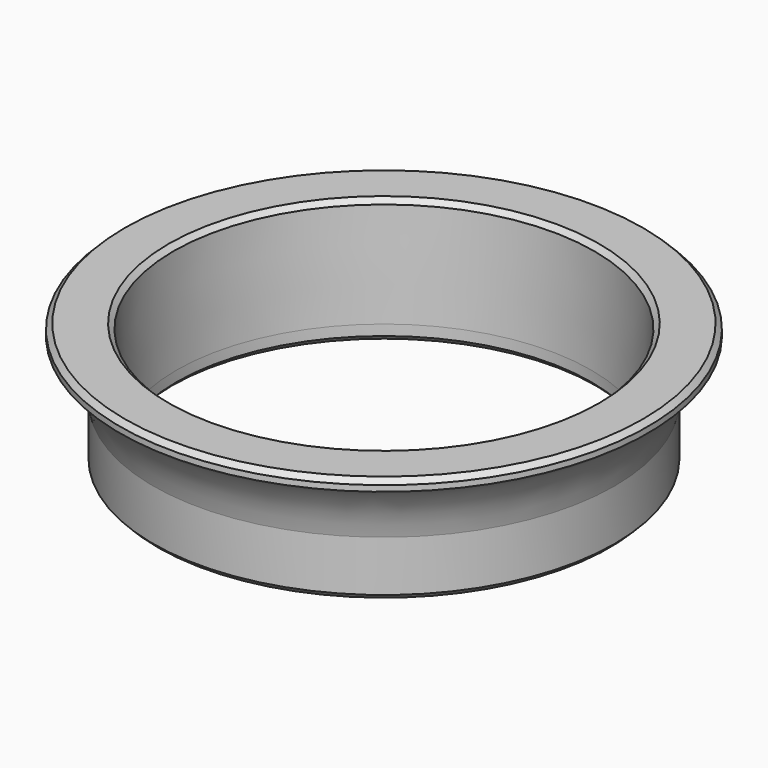
from build123d import *


# Not quite as in the source:
# - a fillet or chamfer that OpenCascade refuses, or shapes differently, is made with other operations: its cross-section is extruded or revolved along the edge and cut away or added


with BuildPart() as f1:
    # F0 (on Front) → F1 (revolve)
    with BuildSketch(Plane.XZ):
        with BuildLine():
            Line((-74.5, 17.9942867992), (-74.5, 0))
            Line((-74.5, 0), (-67, 0))
            Line((-67, 0), (-66.9277426788, 0))
            Line((-66.9277426788, 0), (-66.9277426788, 5))
            Line((-66.9277426788, 5), (-68, 39.9997837721))
            Line((-68, 39.9997837721), (-85.2165701103, 39.9997837721))
            Line((-85.2165701103, 39.9997837721), (-85.2165701103, 36.5022708525))
            add(Edge.make_bspline(
                [(-74.5, 17.9942867992), (-75.2603216112, 22.383891166), (-78.3429778204, 29.8667831773), (-82.1395330633, 34.6033302524), (-85.2165701103, 36.5022708525)],
                knots=[0, 0, 0, 0, 0.533014403, 1, 1, 1, 1], degree=3))
        make_face()
    revolve(axis=Axis((0, 0, 30.7617206126), (0, 0, 1)))

    # F2: chamfer of 1.6 on 4 edges, made by hand

    # F2_s1 → F2_t2 (revolve, cut)
    with BuildSketch(Plane.XZ):
        Polygon((-74.5, 1.6), (-72.9, 0), (-74.5, 0), align=None)
    revolve(axis=Axis((0, 0, 0), (0, 0, 1)), mode=Mode.SUBTRACT)

    # F2_s3 → F2_t4 (revolve, cut)
    with BuildSketch(Plane.XZ):
        Polygon((-68.5277426788, 0), (-66.9277426788, 1.6), (-66.9277426788, 0), align=None)
    revolve(axis=Axis((0, 0, 0), (0, 0, 1)), mode=Mode.SUBTRACT)

    # F2_s5 → F2_t6 (revolve, cut)
    with BuildSketch(Plane.XZ):
        Polygon((-67.9524832296, 38.4487785653), (-69.5517329007, 39.9997837721), (-68, 39.9997837721), align=None)
    revolve(axis=Axis((0, 0, 39.9997837721), (0, 0, 1)), mode=Mode.SUBTRACT)

    # F2_s7 → F2_t8 (revolve, cut)
    with BuildSketch(Plane.XZ):
        Polygon((-83.6165701103, 39.9997837721), (-85.2165701103, 38.3997837721), (-85.2165701103, 39.9997837721), align=None)
    revolve(axis=Axis((0, 0, 39.9997837721), (0, 0, 1)), mode=Mode.SUBTRACT)


solid = f1.part
